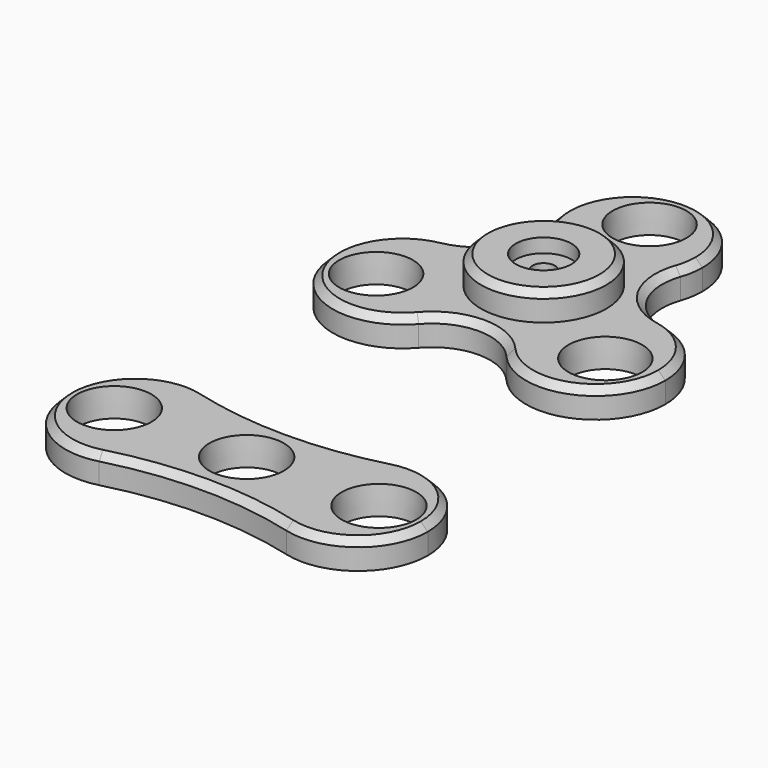
from build123d import *

# Parameters (mm, degrees)
F0_R       = 5.15
F1_DEPTH   = 4
F2_SIZE    = 1
F3_R       = 5.1
F4_DEPTH   = 4
F5_SIZE    = 1
F6_SIZE2   = 3.99999
F6_SIZE    = 0.19999
F6_2_SIZE2 = 3.99999
F6_2_SIZE  = 0.19999
F7_R       = 9
F7_R_2     = 5.29999
F7_R_3     = 4
F8_DEPTH   = 4
F7_R_4     = 1.6
F9_DEPTH   = 2
F10_SIZE   = 1


# Not quite as in the source:
# - a fillet or chamfer is up to 0.001 mm smaller than in the source, because OpenCascade refuses the exact size
# - a feature names something its author has since deleted; it is built from what else it names


with BuildPart() as f1:
    # F0 (on Top) → F1 (new body)
    with BuildSketch(Plane.XY):
        with BuildLine():
            ThreePointArc((-13.4233737216, 9.6623494566), (-8.0701115145, 6.0923614968), (-6, 0))
            ThreePointArc((-6, 0), (-8.0701114601, -6.092361426), (-13.4233735489, -9.6623494106))
            ThreePointArc((-13.4233735489, -9.6623494106), (6.05e-08, -7.903301215), (13.4233736658, -9.6623494417))
            ThreePointArc((13.4233736658, -9.6623494417), (6, -6.16e-08), (13.4233735467, 9.66234941))
            ThreePointArc((13.4233735467, 9.66234941), (-9.05e-08, 7.903301215), (-13.4233737216, 9.6623494566))
        make_face()
        Circle(F0_R, mode=Mode.SUBTRACT)
        with BuildLine():
            ThreePointArc((-13.4233735489, -9.6623494106), (-8.0701114601, -6.092361426), (-6, 0))
            ThreePointArc((-6, 0), (-8.0701115145, 6.0923614968), (-13.4233737216, 9.6623494566))
            ThreePointArc((-13.4233737216, 9.6623494566), (-26, -8.94e-08), (-13.4233735489, -9.6623494106))
        make_face()
        with Locations((-19, 0)):
            Circle(F0_R, mode=Mode.SUBTRACT)
        with BuildLine():
            ThreePointArc((26, 0), (22.0923614251, 7.9298885406), (13.4233735467, 9.66234941))
            ThreePointArc((13.4233735467, 9.66234941), (6, -6.16e-08), (13.4233736658, -9.6623494417))
            ThreePointArc((13.4233736658, -9.6623494417), (22.0923614739, -7.929888503), (26, 0))
        make_face()
        with Locations((19, 0)):
            Circle(F0_R, mode=Mode.SUBTRACT)
    extrude(amount=F1_DEPTH)

    # F2
    f2_edges = [f1.edges().sort_by_distance(p)[0] for p in [
        (0, -7.903301, 4),
    ]]
    chamfer(f2_edges, length=F2_SIZE)

    # F6 (size 0.2 and 4 in the source; OpenCascade refuses exactly that, so slightly less here)
    f6_edges = [f1.edges().sort_by_distance(p)[0] for p in [
        (-24.15, 0, 4),
        (13.85, 0, 4),
        (-5.15, 0, 4),
    ]]
    f6_side = f1.faces().sort_by_distance((0, -6.371888, 4))[0]
    chamfer(f6_edges, length=F6_SIZE, length2=F6_SIZE2, reference=f6_side)


with BuildPart() as f4:
    # F3 (on Top) → F4 (new body)
    with BuildSketch(Plane.XY):
        with BuildLine():
            ThreePointArc((9.4491118238, 66.0191849315), (9.8613162975, 67.632802458), (10, 69.292453289))
            ThreePointArc((10, 69.292453289), (-1.6596509098, 79.1537695733), (-9.4491117716, 66.0191847805))
            ThreePointArc((-9.4491117716, 66.0191847805), (7.99e-08, 59.292453289), (9.4491118238, 66.0191849315))
        make_face()
        with Locations((0, 72.292453289)):
            Circle(F3_R, mode=Mode.SUBTRACT)
        with BuildLine():
            ThreePointArc((9.4491118238, 66.0191849315), (7.99e-08, 59.292453289), (-9.4491117716, 66.0191847805))
            ThreePointArc((-9.4491117716, 66.0191847805), (-10.1062544883, 59.1273014814), (-15.7462296119, 55.1122581983))
            ThreePointArc((-15.7462296119, 55.1122581983), (-7.4884488411, 53.0027785582), (-3.8564064606, 45.292453289))
            ThreePointArc((-3.8564064606, 45.292453289), (-4.4864305642, 41.7990950622), (-6.2971168007, 38.7459168125))
            ThreePointArc((-6.2971168007, 38.7459168125), (1.374e-07, 41.6227560689), (6.2971169806, 38.7459166047))
            ThreePointArc((6.2971169806, 38.7459166047), (5.1961526478, 50.2924536788), (15.74622968, 55.1122581852))
            ThreePointArc((15.74622968, 55.1122581852), (10.1062544657, 59.1273015205), (9.4491118238, 66.0191849315))
        make_face()
        with Locations((0, 53.292453289)):
            Circle(F3_R, mode=Mode.SUBTRACT)
        with BuildLine():
            ThreePointArc((23.8564064606, 45.292453289), (21.5667317518, 51.6604108818), (15.74622968, 55.1122581852))
            ThreePointArc((15.74622968, 55.1122581852), (5.1961526478, 50.2924536788), (6.2971169806, 38.7459166047))
            ThreePointArc((6.2971169806, 38.7459166047), (17.3497648161, 35.9224774406), (23.8564064606, 45.292453289))
        make_face()
        with Locations((16.4544826719, 43.792453289)):
            Circle(F3_R, mode=Mode.SUBTRACT)
        with BuildLine():
            ThreePointArc((-3.8564064606, 45.292453289), (-7.4884488411, 53.0027785582), (-15.7462296119, 55.1122581983))
            ThreePointArc((-15.7462296119, 55.1122581983), (-22.516660222, 40.2924528103), (-6.2971168007, 38.7459168125))
            ThreePointArc((-6.2971168007, 38.7459168125), (-4.4864305642, 41.7990950622), (-3.8564064606, 45.292453289))
        make_face()
        with Locations((-16.4544826719, 43.792453289)):
            Circle(F3_R, mode=Mode.SUBTRACT)
    extrude(amount=F4_DEPTH)

    # F5
    f5_edges = [f4.edges().sort_by_distance(p)[0] for p in [
        (-22.51666, 40.292453, 4),
    ]]
    chamfer(f5_edges, length=F5_SIZE)

    # F6#2 (size 0.2 and 4 in the source; OpenCascade refuses exactly that, so slightly less here)
    f6_2_edges = [f4.edges().sort_by_distance(p)[0] for p in [
        (-21.554483, 43.792453, 4),
        (-5.1, 53.292453, 4),
        (-5.1, 72.292453, 4),
        (11.354483, 43.792453, 4),
    ]]
    f6_2_side = f4.faces().sort_by_distance((-21.113025, 41.102842, 4))[0]
    chamfer(f6_2_edges, length=F6_2_SIZE, length2=F6_2_SIZE2, reference=f6_2_side)


with BuildPart() as f8:
    # F7 (on face) → F8 (new body)
    with BuildSketch(Plane.XY.offset(4)):
        with Locations((0, 53.292453289)):
            Circle(F7_R)
        with Locations((0, 53.292453289)):
            Circle(F7_R_2, mode=Mode.SUBTRACT)
        with Locations((0, 53.292453289)):
            Circle(F7_R_2)
        with Locations((0, 53.292453289)):
            Circle(F7_R_3, mode=Mode.SUBTRACT)
    extrude(amount=F8_DEPTH)

    # F7 (on face) → F9 (join)
    with BuildSketch(Plane.XY.offset(4)):
        with Locations((0, 53.292453289)):
            Circle(F7_R_3)
        with Locations((0, 53.292453289)):
            Circle(F7_R_4, mode=Mode.SUBTRACT)
    extrude(amount=F9_DEPTH)

    # F10
    f10_edges = [f8.edges().sort_by_distance(p)[0] for p in [
        (-9, 53.292453, 8),
    ]]
    chamfer(f10_edges, length=F10_SIZE)


solid = Compound([f1.part, f4.part, f8.part])
